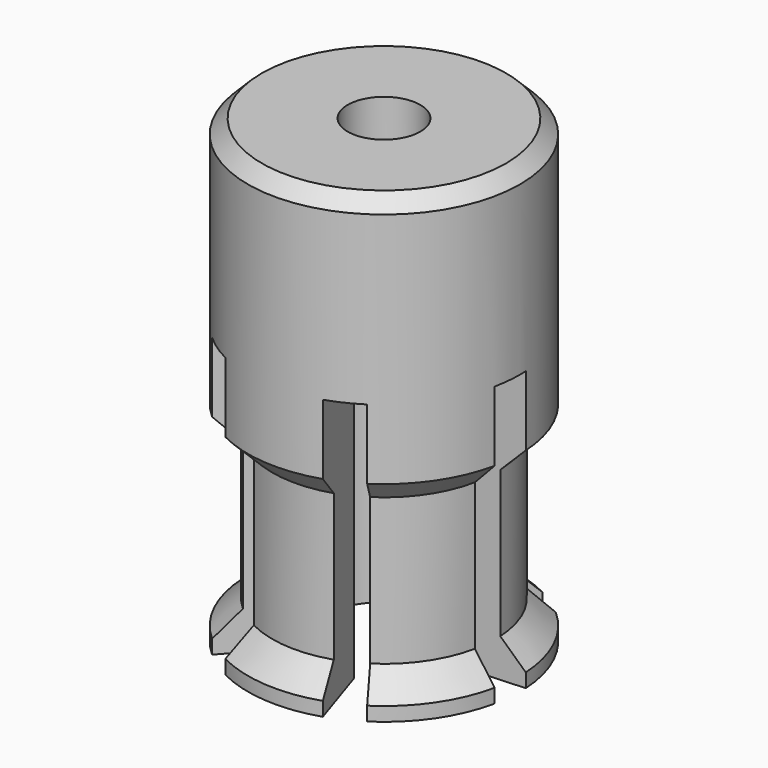
from build123d import *

# Parameters (mm, degrees)
F0_R          = 9.75
F0_R_2        = 4.75
F0_R_3        = 2.6
F1_DEPTH      = 10
F2_DEPTH      = 10
F3_R          = 8
F3_R_2        = 4.75
F4_DEPTH      = 10
F5_R          = 9.75
F5_R_2        = 8
F5_R_3        = 4.75
F6_DEPTH      = 3
F7_S5_R       = 8
F7_T6_DEPTH   = 15
F9_DEPTH      = 20
F11_D         = 5
F11_DEPTH     = 14
F11_TIP       = 1.5021515476
F12_SIZE      = 1
F13_T4_ANGLE  = 45
F13_S5_R      = 8
F13_T6_DEPTH  = 17
F13_T10_ANGLE = 45
F13_S11_R     = 8
F13_T12_DEPTH = 17
F13_T16_ANGLE = 45
F13_S17_R     = 8
F13_T18_DEPTH = 17
F13_T22_ANGLE = 45
F13_S23_R     = 8
F13_T24_DEPTH = 17
F13_T28_ANGLE = 45
F13_S29_R     = 8
F13_T30_DEPTH = 17
F13_T34_ANGLE = 45
F13_S35_R     = 8
F13_T36_DEPTH = 17


# Not quite as in the source:
# - a fillet or chamfer that OpenCascade refuses, or shapes differently, is made with other operations: its cross-section is extruded or revolved along the edge and cut away or added


with BuildPart() as f1:
    # F0 (on Top) → F1 (new body)
    with BuildSketch(Plane.XY):
        with Locations((0, -2.0069764376)):
            Circle(F0_R)
        with Locations((0, -2.0069764376)):
            Circle(F0_R_2, mode=Mode.SUBTRACT)
        with Locations((0, -2.0069764376)):
            Circle(F0_R_2)
        with Locations((0, -2.0069764376)):
            Circle(F0_R_3, mode=Mode.SUBTRACT)
    extrude(amount=F1_DEPTH)

    # F0 (on Top) → F2 (join)
    with BuildSketch(Plane.XY):
        with Locations((0, -2.0069764376)):
            Circle(F0_R)
        with Locations((0, -2.0069764376)):
            Circle(F0_R_2, mode=Mode.SUBTRACT)
    extrude(amount=-F2_DEPTH)

    # F3 (on face) → F4 (join)
    with BuildSketch(Plane(origin=(0, 0, -10), x_dir=(1, 0, 0), z_dir=(0, 0, -1))):
        with Locations((0, 2.0069764376)):
            Circle(F3_R)
        with Locations((0, 2.0069764376)):
            Circle(F3_R_2, mode=Mode.SUBTRACT)
    extrude(amount=F4_DEPTH)

    # F5 (on face) → F6 (join)
    with BuildSketch(Plane(origin=(0, 0, -20), x_dir=(1, 0, 0), z_dir=(0, 0, -1))):
        with Locations((0, 2.0069764376)):
            Circle(F5_R)
        with Locations((0, 2.0069764376)):
            Circle(F5_R_2, mode=Mode.SUBTRACT)
        with Locations((0, 2.0069764376)):
            Circle(F5_R_2)
        with Locations((0, 2.0069764376)):
            Circle(F5_R_3, mode=Mode.SUBTRACT)
    extrude(amount=F6_DEPTH)

    # F7: chamfer of 2 on 1 edges, made by hand


with BuildPart() as f7_tool2:
    # F7_s3 → F7_t4 (revolve)
    with BuildSketch(Plane.XZ.offset(2.0069764376)):
        Polygon((7.75, -20), (9.75, -22), (9.75, -20), align=None)
    revolve(axis=Axis((0, -2.0069764376, -20), (0, 0, -1)))

    # F7_s5 → F7_t6 (cut, symmetric)
    with BuildSketch(Plane.XY.offset(-21)):
        with Locations((0, -2.0069764376)):
            Circle(F7_S5_R)
    extrude(amount=F7_T6_DEPTH, both=True, mode=Mode.SUBTRACT)


with BuildPart() as f1_1:
    add(f1.part)

    # F7_t1: cut F7_tool2
    add(f7_tool2.part, mode=Mode.SUBTRACT)

    # F8 (on face) → F9 (cut)
    with BuildSketch(Plane(origin=(0, 0, -23), x_dir=(1, 0, 0), z_dir=(0, 0, -1))):
        with BuildLine():
            ThreePointArc((-1.4773760244, -2.5074294018), (-2.053985072, -2.2759717671), (-2.5954498656, -1.9712317011))
            Line((-2.5954498656, -1.9712317011), (-5.3275023558, -6.1588192156))
            ThreePointArc((-5.3275023558, -6.1588192156), (-4.2160746215, -6.7843382983), (-3.0325086816, -7.2594355485))
            Line((-3.0325086816, -7.2594355485), (-1.4773760244, -2.5074294018))
        make_face()
        with BuildLine():
            Line((6.5086938411, -5.252459111), (3.1709021277, -1.5296716502))
            ThreePointArc((3.1709021277, -1.5296716502), (2.6821494123, -1.9133009161), (2.1475043769, -2.2298531497))
            Line((2.1475043769, -2.2298531497), (4.4080352999, -6.6896737678))
            ThreePointArc((4.4080352999, -6.6896737678), (5.5054645832, -6.0399086569), (6.5086938411, -5.252459111))
        make_face()
        with BuildLine():
            Line((9.5412025227, 4.0139528751), (4.6482781521, 2.9847341892))
            ThreePointArc((4.6482781521, 2.9847341892), (4.7245010965, 2.4984938725), (4.75, 2.0069764376))
            ThreePointArc((4.75, 2.0069764376), (4.7482382339, 1.8776177344), (4.7429542425, 1.748354989))
            Line((4.7429542425, 1.748354989), (9.7355376556, 1.4761218853))
            ThreePointArc((9.7355376556, 1.4761218853), (9.7463837433, 1.7414506784), (9.75, 2.0069764376))
            ThreePointArc((9.75, 2.0069764376), (9.6976601455, 3.015880646), (9.5412025227, 4.0139528751))
        make_face()
        with BuildLine():
            Line((3.0325086816, 11.2733884237), (1.4773760244, 6.5213822769))
            ThreePointArc((1.4773760244, 6.5213822769), (2.053985072, 6.2899246422), (2.5954498656, 5.9851845763))
            Line((2.5954498656, 5.9851845763), (5.3275023558, 10.1727720907))
            ThreePointArc((5.3275023558, 10.1727720907), (4.2160746215, 10.7982911735), (3.0325086816, 11.2733884237))
        make_face()
        with BuildLine():
            Line((-6.5086938411, 9.2664119861), (-3.1709021277, 5.5436245253))
            ThreePointArc((-3.1709021277, 5.5436245253), (-2.6821494123, 5.9272537913), (-2.1475043769, 6.2438060248))
            Line((-2.1475043769, 6.2438060248), (-4.4080352999, 10.703626643))
            ThreePointArc((-4.4080352999, 10.703626643), (-5.5054645832, 10.053861532), (-6.5086938411, 9.2664119861))
        make_face()
        with BuildLine():
            Line((-9.5412025227, 0), (-4.6482781521, 1.0292186859))
            ThreePointArc((-4.6482781521, 1.0292186859), (-4.7361344844, 1.6443055866), (-4.7429542425, 2.2655978861))
            Line((-4.7429542425, 2.2655978861), (-9.7355376556, 2.5378309898))
            ThreePointArc((-9.7355376556, 2.5378309898), (-9.7215392047, 1.2625467961), (-9.5412025227, 0))
        make_face()
    extrude(amount=-F9_DEPTH, mode=Mode.SUBTRACT)

    # F11 (one way)
    with BuildSketch(Plane.XZ):
        with Locations((0, 5)):
            Circle(F11_D / 2)
    extrude(amount=-F11_DEPTH, mode=Mode.SUBTRACT)
    with Locations(Plane.XZ):
        with Locations((0, 5)):
            with Locations((0, 0, -(F11_DEPTH + F11_TIP / 2))):  # 118° drill point
                Cone(0, F11_D / 2, F11_TIP, mode=Mode.SUBTRACT)

    # F12
    f12_edges = [f1_1.edges().sort_by_distance(p)[0] for p in [
        (-9.75, -2.006976, 10),
    ]]
    chamfer(f12_edges, length=F12_SIZE)

    # F13: chamfer of 2 on 6 edges, made by hand


with BuildPart() as f13_tool2:
    # F13_s3 → F13_t4 (revolve)
    with BuildSketch(Plane(origin=(0.8093383291, -0.4102259882, 0), x_dir=(0, 0, 1), z_dir=(0.8919641236, -0.4521061846, 0))):
        with BuildLine():
            Line((-7.9434314575, -8.0164175632), (-10.0565685425, -5.9032804782))
            Line((-10.0565685425, -5.9032804782), (-10.0965685425, -5.9032804782))
            ThreePointArc((-10.0965685425, -5.9032804782), (-10.04, -6.9315647495), (-10.04, -7.9598490207))
            Line((-10.04, -7.9598490207), (-10, -7.9998490207))
            ThreePointArc((-10, -7.9998490207), (-8.9717157288, -7.9998490207), (-7.9434314575, -8.0564175632))
            Line((-7.9434314575, -8.0564175632), (-7.9434314575, -8.0164175632))
        make_face()
    revolve(axis=Axis((0, -2.0069764376, -10), (0, 0, 1)), revolution_arc=F13_T4_ANGLE)

    # F13_s5 → F13_t6 (cut, symmetric)
    with BuildSketch(Plane.XY.offset(-9.5)):
        with Locations((0, -2.0069764376)):
            Circle(F13_S5_R)
    extrude(amount=F13_T6_DEPTH, both=True, mode=Mode.SUBTRACT)


with BuildPart() as f1_2:
    add(f1_1.part)

    # F13_t1: cut F13_tool2
    add(f13_tool2.part, mode=Mode.SUBTRACT)


with BuildPart() as f13_tool8:
    # F13_s9 → F13_t10 (revolve)
    with BuildSketch(Plane(origin=(-0.9184493274, -0.5992117808, 0), x_dir=(0, 0, 1), z_dir=(0.8375175029, 0.546410498, 0))):
        with BuildLine():
            Line((-7.9434314575, -8.1256906481), (-10.0565685425, -6.0125535632))
            Line((-10.0565685425, -6.0125535632), (-10.0965685425, -6.0125535632))
            ThreePointArc((-10.0965685425, -6.0125535632), (-10.04, -7.0408378344), (-10.04, -8.0691221057))
            Line((-10.04, -8.0691221057), (-10, -8.1091221057))
            ThreePointArc((-10, -8.1091221057), (-8.9717157288, -8.1091221057), (-7.9434314575, -8.1656906481))
            Line((-7.9434314575, -8.1656906481), (-7.9434314575, -8.1256906481))
        make_face()
    revolve(axis=Axis((0, -2.0069764376, -10), (0, 0, 1)), revolution_arc=F13_T10_ANGLE)

    # F13_s11 → F13_t12 (cut, symmetric)
    with BuildSketch(Plane.XY.offset(-9.5)):
        with Locations((0, -2.0069764376)):
            Circle(F13_S11_R)
    extrude(amount=F13_T12_DEPTH, both=True, mode=Mode.SUBTRACT)


with BuildPart() as f1_3:
    add(f1_2.part)

    # F13_t7: cut F13_tool8
    add(f13_tool8.part, mode=Mode.SUBTRACT)


with BuildPart() as f13_tool14:
    # F13_s15 → F13_t16 (revolve)
    with BuildSketch(Plane(origin=(0.1091109983, -2.0010268874, 0), x_dir=(0, 0, 1), z_dir=(0.0544466207, -0.9985166826, 0))):
        with BuildLine():
            Line((-7.9434314575, -9.6972954576), (-10.0565685425, -7.5841583726))
            Line((-10.0565685425, -7.5841583726), (-10.0965685425, -7.5841583726))
            ThreePointArc((-10.0965685425, -7.5841583726), (-10.04, -8.6124426438), (-10.04, -9.6407269151))
            Line((-10.04, -9.6407269151), (-10, -9.6807269151))
            ThreePointArc((-10, -9.6807269151), (-8.9717157288, -9.6807269151), (-7.9434314575, -9.7372954576))
            Line((-7.9434314575, -9.7372954576), (-7.9434314575, -9.6972954576))
        make_face()
    revolve(axis=Axis((0, -2.0069764376, -10), (0, 0, 1)), revolution_arc=F13_T16_ANGLE)

    # F13_s17 → F13_t18 (cut, symmetric)
    with BuildSketch(Plane.XY.offset(-9.5)):
        with Locations((0, -2.0069764376)):
            Circle(F13_S17_R)
    extrude(amount=F13_T18_DEPTH, both=True, mode=Mode.SUBTRACT)


with BuildPart() as f1_4:
    add(f1_3.part)

    # F13_t13: cut F13_tool14
    add(f13_tool14.part, mode=Mode.SUBTRACT)


with BuildPart() as f13_tool20:
    # F13_s21 → F13_t22 (revolve)
    with BuildSketch(Plane(origin=(-0.9184493274, -0.5992117808, 0), x_dir=(0, 0, 1), z_dir=(-0.8375175029, -0.546410498, 0))):
        with BuildLine():
            Line((-7.9434314575, -11.4874464368), (-10.0565685425, -9.3743093519))
            Line((-10.0565685425, -9.3743093519), (-10.0965685425, -9.3743093519))
            ThreePointArc((-10.0965685425, -9.3743093519), (-10.04, -10.4025936231), (-10.04, -11.4308778943))
            Line((-10.04, -11.4308778943), (-10, -11.4708778943))
            ThreePointArc((-10, -11.4708778943), (-8.9717157288, -11.4708778943), (-7.9434314575, -11.5274464368))
            Line((-7.9434314575, -11.5274464368), (-7.9434314575, -11.4874464368))
        make_face()
    revolve(axis=Axis((0, -2.0069764376, -10), (0, 0, 1)), revolution_arc=F13_T22_ANGLE)

    # F13_s23 → F13_t24 (cut, symmetric)
    with BuildSketch(Plane.XY.offset(-9.5)):
        with Locations((0, -2.0069764376)):
            Circle(F13_S23_R)
    extrude(amount=F13_T24_DEPTH, both=True, mode=Mode.SUBTRACT)


with BuildPart() as f1_5:
    add(f1_4.part)

    # F13_t19: cut F13_tool20
    add(f13_tool20.part, mode=Mode.SUBTRACT)


with BuildPart() as f13_tool26:
    # F13_s27 → F13_t28 (revolve)
    with BuildSketch(Plane(origin=(0.8093383291, -0.4102259882, 0), x_dir=(0, 0, 1), z_dir=(-0.8919641236, 0.4521061846, 0))):
        with BuildLine():
            Line((-7.9434314575, -11.5967195218), (-10.0565685425, -9.4835824368))
            Line((-10.0565685425, -9.4835824368), (-10.0965685425, -9.4835824368))
            ThreePointArc((-10.0965685425, -9.4835824368), (-10.04, -10.511866708), (-10.04, -11.5401509793))
            Line((-10.04, -11.5401509793), (-10, -11.5801509793))
            ThreePointArc((-10, -11.5801509793), (-8.9717157288, -11.5801509793), (-7.9434314575, -11.6367195218))
            Line((-7.9434314575, -11.6367195218), (-7.9434314575, -11.5967195218))
        make_face()
    revolve(axis=Axis((0, -2.0069764376, -10), (0, 0, 1)), revolution_arc=F13_T28_ANGLE)

    # F13_s29 → F13_t30 (cut, symmetric)
    with BuildSketch(Plane.XY.offset(-9.5)):
        with Locations((0, -2.0069764376)):
            Circle(F13_S29_R)
    extrude(amount=F13_T30_DEPTH, both=True, mode=Mode.SUBTRACT)


with BuildPart() as f1_6:
    add(f1_5.part)

    # F13_t25: cut F13_tool26
    add(f13_tool26.part, mode=Mode.SUBTRACT)


with BuildPart() as f13_tool32:
    # F13_s33 → F13_t34 (revolve)
    with BuildSketch(Plane(origin=(0.1091109983, -2.0010268874, 0), x_dir=(0, 0, 1), z_dir=(-0.0544466207, 0.9985166826, 0))):
        with BuildLine():
            Line((-7.9434314575, -9.9158416274), (-10.0565685425, -7.8027045424))
            Line((-10.0565685425, -7.8027045424), (-10.0965685425, -7.8027045424))
            ThreePointArc((-10.0965685425, -7.8027045424), (-10.04, -8.8309888137), (-10.04, -9.8592730849))
            Line((-10.04, -9.8592730849), (-10, -9.8992730849))
            ThreePointArc((-10, -9.8992730849), (-8.9717157288, -9.8992730849), (-7.9434314575, -9.9558416274))
            Line((-7.9434314575, -9.9558416274), (-7.9434314575, -9.9158416274))
        make_face()
    revolve(axis=Axis((0, -2.0069764376, -10), (0, 0, 1)), revolution_arc=F13_T34_ANGLE)

    # F13_s35 → F13_t36 (cut, symmetric)
    with BuildSketch(Plane.XY.offset(-9.5)):
        with Locations((0, -2.0069764376)):
            Circle(F13_S35_R)
    extrude(amount=F13_T36_DEPTH, both=True, mode=Mode.SUBTRACT)


with BuildPart() as f1_7:
    add(f1_6.part)

    # F13_t31: cut F13_tool32
    add(f13_tool32.part, mode=Mode.SUBTRACT)


solid = f1_7.part
